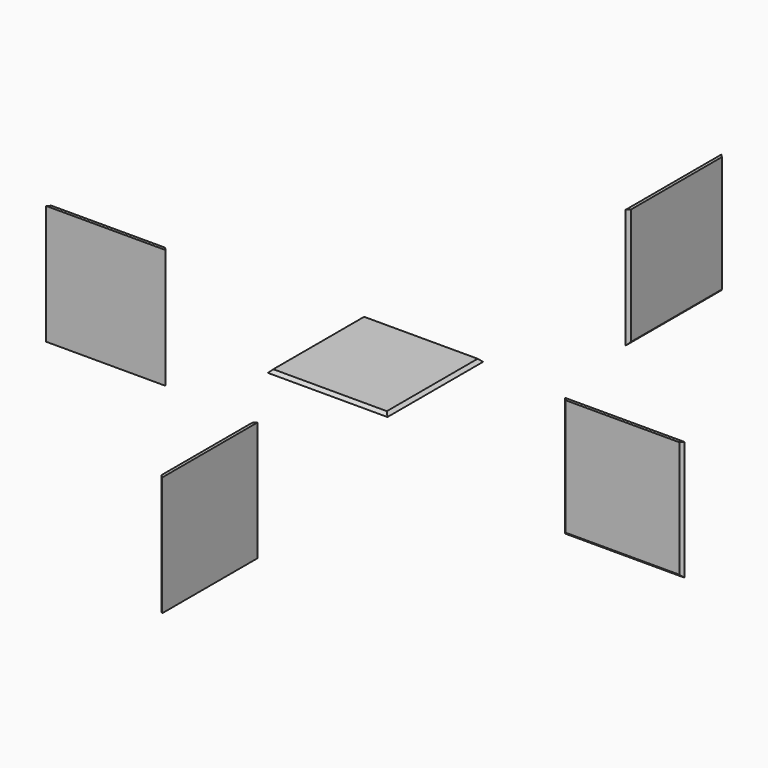
from build123d import *

# Parameters (mm, degrees)
F0_W       = 200
F0_H       = 200
F1_DEPTH   = 5
F2_SIZE    = 4.99999
F3_W       = 200
F3_H       = 200
F4_DEPTH   = 5
F5_SIZE    = 4.99999
F6_W       = 200
F6_H       = 200
F7_DEPTH   = 5
F8_SIZE    = 4.99999
F9_W       = 200
F9_H       = 200
F10_DEPTH  = 5
F11_SIZE   = 4.99999
F11_2_SIZE = 4.99999


# Not quite as in the source:
# - a fillet or chamfer is up to 0.001 mm smaller than in the source, because OpenCascade refuses the exact size


with BuildPart() as f1:
    # F0 (on Top) → F1 (new body)
    with BuildSketch(Plane.XY):
        with Locations((-45.1127041131, -19.84155476)):
            Rectangle(F0_W, F0_H)
    extrude(amount=F1_DEPTH)

    # F2 (size 5 in the source; OpenCascade refuses exactly that, so slightly less here)
    f2_edges = [f1.edges().sort_by_distance(p)[0] for p in [
        (-45.112704, -119.841555, 5),
        (54.887296, -19.841555, 5),
        (-45.112704, 80.158445, 5),
        (-145.112704, -19.841555, 5),
    ]]
    chamfer(f2_edges, length=F2_SIZE)


with BuildPart() as f4:
    # F3 (on Front) → F4 (new body)
    with BuildSketch(Plane.XZ):
        with Locations((356.2874466181, -54.8991493524)):
            Rectangle(F3_W, F3_H)
    extrude(amount=F4_DEPTH)

    # F5 (size 5 in the source; OpenCascade refuses exactly that, so slightly less here)
    f5_edges = [f4.edges().sort_by_distance(p)[0] for p in [
        (356.287447, -5, -154.899149),
        (256.287447, -5, -54.899149),
        (456.287447, -5, -54.899149),
    ]]
    chamfer(f5_edges, length=F5_SIZE)


with BuildPart() as f7:
    # F6 (on Front) → F7 (new body)
    with BuildSketch(Plane.XZ):
        with Locations((-508.1502228975, -51.3473520487)):
            Rectangle(F6_W, F6_H)
    extrude(amount=F7_DEPTH)

    # F8 (size 5 in the source; OpenCascade refuses exactly that, so slightly less here)
    f8_edges = [f7.edges().sort_by_distance(p)[0] for p in [
        (-408.150223, 0, -51.347352),
        (-508.150223, 0, -151.347352),
        (-608.150223, 0, -51.347352),
    ]]
    chamfer(f8_edges, length=F8_SIZE)


with BuildPart() as f10:
    # F9 (on Right) → F10 (new body)
    with BuildSketch(Plane.YZ):
        with Locations((547.0643907785, -42.9269958158)):
            Rectangle(F9_W, F9_H)
    extrude(amount=F10_DEPTH)

    # F11 (size 5 in the source; OpenCascade refuses exactly that, so slightly less here)
    f11_edges = [f10.edges().sort_by_distance(p)[0] for p in [
        (5, 447.064391, -42.926996),
        (5, 547.064391, -142.926996),
        (5, 647.064391, -42.926996),
    ]]
    chamfer(f11_edges, length=F11_SIZE)


with BuildPart() as f10b:
    # F9 (on Right) → F10, piece 2 (new body)
    with BuildSketch(Plane.YZ):
        with Locations((-429.2863249779, -39.0882730484)):
            Rectangle(F9_W, F9_H)
    extrude(amount=F10_DEPTH)

    # F11#2 (size 5 in the source; OpenCascade refuses exactly that, so slightly less here)
    f11_2_edges = [f10b.edges().sort_by_distance(p)[0] for p in [
        (0, -329.286325, -39.088273),
        (0, -429.286325, -139.088273),
        (0, -529.286325, -39.088273),
    ]]
    chamfer(f11_2_edges, length=F11_2_SIZE)


solid = Compound([f1.part, f4.part, f7.part, f10.part, f10b.part])
